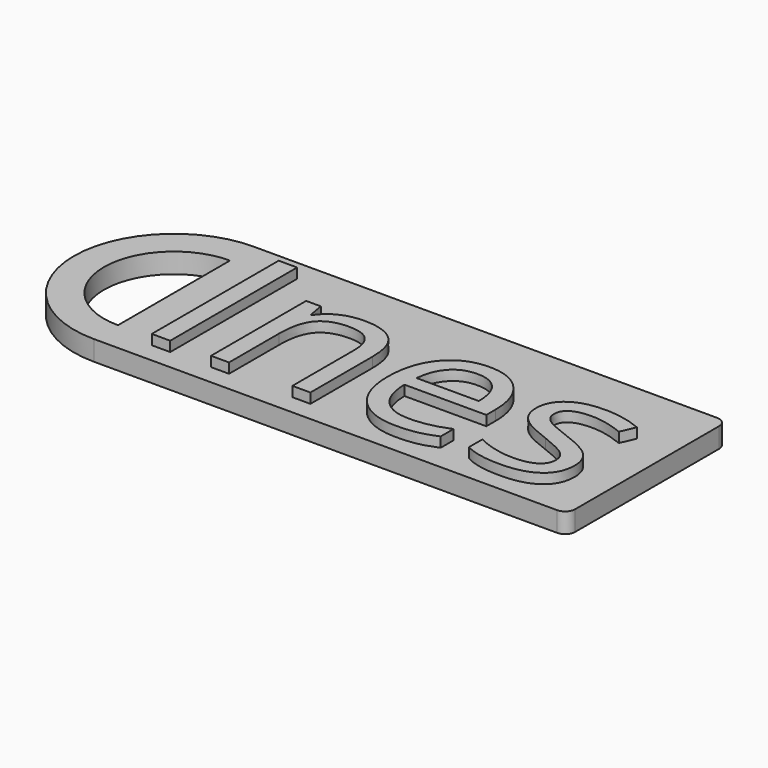
from build123d import *

# Parameters (mm, degrees)
F0_W         = 1.84375
F0_H         = 15.8645833333
F0_TEXT_SIZE = 22.2222222222
F1_DEPTH     = 2
F2_DEPTH     = 3
F3_R         = 1


# Not quite as in the source:
# - Text() gives the source's letters only with a copy of the font that has no kerning and outlines rounded to 1/6400 em; it was checked with that copy


with BuildPart() as f1:
    # F0 (on Top) → F1 (new body)
    with BuildSketch(Plane.XY):
        Polygon((28.77725482, 9.7942796086), (-18.5456618466, 9.7942796086), (-18.5456618466, 6.7942796086), (-18.5456618466, -7.2057203914), (-18.5456618466, -10.2057203914), (28.77725482, -10.2057203914), align=None)
        with Locations((-13.4432312911, -0.2734287247)):
            Rectangle(F0_W, F0_H, mode=Mode.SUBTRACT)
        with BuildLine():
            Line((1.4994770423, -8.2057203914), (-0.3026062911, -8.2057203914))
            Line((-0.3026062911, -8.2057203914), (-0.3026062911, -0.5112759469))
            add(Edge.make_bspline(
                [(-0.3026062911, -0.5112759469), (-0.3026062911, 0.940112942), (-0.9640646244, 1.6571268309)],
                knots=[0, 0, 0, 1, 1, 1], degree=2))
            add(Edge.make_bspline(
                [(-0.9640646244, 1.6571268309), (-1.6255229577, 2.3741407197), (-3.0387174022, 2.3741407197)],
                knots=[0, 0, 0, 1, 1, 1], degree=2))
            add(Edge.make_bspline(
                [(-3.0387174022, 2.3741407197), (-4.9033007355, 2.3741407197), (-5.7713562911, 1.3654601642)],
                knots=[0, 0, 0, 1, 1, 1], degree=2))
            add(Edge.make_bspline(
                [(-5.7713562911, 1.3654601642), (-6.6394118466, 0.3567796086), (-6.6394118466, -1.966137058)],
                knots=[0, 0, 0, 1, 1, 1], degree=2))
            Line((-6.6394118466, -1.966137058), (-6.6394118466, -8.2057203914))
            Line((-6.6394118466, -8.2057203914), (-8.44149518, -8.2057203914))
            Line((-8.44149518, -8.2057203914), (-8.44149518, 3.6866407197))
            Line((-8.44149518, 3.6866407197), (-6.9762174022, 3.6866407197))
            Line((-6.9762174022, 3.6866407197), (-6.6845507355, 2.0581684975))
            Line((-6.6845507355, 2.0581684975), (-6.59774518, 2.0581684975))
            add(Edge.make_bspline(
                [(-6.59774518, 2.0581684975), (-6.0421896244, 2.9366407197), (-5.0439257355, 3.4210157197)],
                knots=[0, 0, 0, 1, 1, 1], degree=2))
            add(Edge.make_bspline(
                [(-5.0439257355, 3.4210157197), (-4.0456618466, 3.9053907197), (-2.8199674022, 3.9053907197)],
                knots=[0, 0, 0, 1, 1, 1], degree=2))
            add(Edge.make_bspline(
                [(-2.8199674022, 3.9053907197), (-0.6706618466, 3.9053907197), (0.4144075978, 2.8689323864)],
                knots=[0, 0, 0, 1, 1, 1], degree=2))
            add(Edge.make_bspline(
                [(0.4144075978, 2.8689323864), (1.4994770423, 1.8324740531), (1.4994770423, -0.4487759469)],
                knots=[0, 0, 0, 1, 1, 1], degree=2))
            Line((1.4994770423, -0.4487759469), (1.4994770423, -8.2057203914))
        make_face(mode=Mode.SUBTRACT)
        with BuildLine():
            add(Edge.make_bspline(
                [(12.27725482, -8.2439148358), (11.4265603756, -8.4244703914), (10.2216992645, -8.4244703914)],
                knots=[0, 0, 0, 1, 1, 1], degree=2))
            add(Edge.make_bspline(
                [(10.2216992645, -8.4244703914), (7.5862825978, -8.4244703914), (6.0602409311, -6.8168315025)],
                knots=[0, 0, 0, 1, 1, 1], degree=2))
            add(Edge.make_bspline(
                [(6.0602409311, -6.8168315025), (4.5341992645, -5.2091926136), (4.5341992645, -2.3584981691)],
                knots=[0, 0, 0, 1, 1, 1], degree=2))
            add(Edge.make_bspline(
                [(4.5341992645, -2.3584981691), (4.5341992645, 0.5199740531), (5.9508659311, 2.2126823864)],
                knots=[0, 0, 0, 1, 1, 1], degree=2))
            add(Edge.make_bspline(
                [(5.9508659311, 2.2126823864), (7.3675325978, 3.9053907197), (9.7564214867, 3.9053907197)],
                knots=[0, 0, 0, 1, 1, 1], degree=2))
            add(Edge.make_bspline(
                [(9.7564214867, 3.9053907197), (11.9890603756, 3.9053907197), (13.2911437089, 2.4349046086)],
                knots=[0, 0, 0, 1, 1, 1], degree=2))
            add(Edge.make_bspline(
                [(13.2911437089, 2.4349046086), (14.5932270423, 0.9644184975), (14.5932270423, -1.4453037247)],
                knots=[0, 0, 0, 1, 1, 1], degree=2))
            Line((14.5932270423, -1.4453037247), (14.5932270423, -2.5841926136))
            Line((14.5932270423, -2.5841926136), (6.40225482, -2.5841926136))
            add(Edge.make_bspline(
                [(6.40225482, -2.5841926136), (6.4578103756, -4.6779426136), (7.4612825978, -5.763012058)],
                knots=[0, 0, 0, 1, 1, 1], degree=2))
            add(Edge.make_bspline(
                [(7.4612825978, -5.763012058), (8.46475482, -6.8480815025), (10.2876714867, -6.8480815025)],
                knots=[0, 0, 0, 1, 1, 1], degree=2))
            add(Edge.make_bspline(
                [(10.2876714867, -6.8480815025), (12.2078103756, -6.8480815025), (14.0828103756, -6.0459981691)],
                knots=[0, 0, 0, 1, 1, 1], degree=2))
            Line((14.0828103756, -6.0459981691), (14.0828103756, -7.653637058))
            add(Edge.make_bspline(
                [(14.0828103756, -7.653637058), (13.1279492645, -8.0633592803), (12.27725482, -8.2439148358)],
                knots=[0, 0, 0, 1, 1, 1], degree=2))
        make_face(mode=Mode.SUBTRACT)
        with BuildLine():
            add(Edge.make_bspline(
                [(24.5932270423, -2.997387058), (25.3362825978, -3.778637058), (25.3362825978, -4.9626648358)],
                knots=[0, 0, 0, 1, 1, 1], degree=2))
            add(Edge.make_bspline(
                [(25.3362825978, -4.9626648358), (25.3362825978, -6.622387058), (24.1001714867, -7.5234287247)],
                knots=[0, 0, 0, 1, 1, 1], degree=2))
            add(Edge.make_bspline(
                [(24.1001714867, -7.5234287247), (22.8640603756, -8.4244703914), (20.6279492645, -8.4244703914)],
                knots=[0, 0, 0, 1, 1, 1], degree=2))
            add(Edge.make_bspline(
                [(20.6279492645, -8.4244703914), (18.2633659311, -8.4244703914), (16.9404492645, -7.6744703914)],
                knots=[0, 0, 0, 1, 1, 1], degree=2))
            Line((16.9404492645, -7.6744703914), (16.9404492645, -6.0043315025))
            add(Edge.make_bspline(
                [(16.9404492645, -6.0043315025), (17.7980881534, -6.4383592803), (18.7789909311, -6.6866231691)],
                knots=[0, 0, 0, 1, 1, 1], degree=2))
            add(Edge.make_bspline(
                [(18.7789909311, -6.6866231691), (19.7598937089, -6.934887058), (20.6730881534, -6.934887058)],
                knots=[0, 0, 0, 1, 1, 1], degree=2))
            add(Edge.make_bspline(
                [(20.6730881534, -6.934887058), (22.0828103756, -6.934887058), (22.8414909311, -6.4852342803)],
                knots=[0, 0, 0, 1, 1, 1], degree=2))
            add(Edge.make_bspline(
                [(22.8414909311, -6.4852342803), (23.6001714867, -6.0355815025), (23.6001714867, -5.1119703914)],
                knots=[0, 0, 0, 1, 1, 1], degree=2))
            add(Edge.make_bspline(
                [(23.6001714867, -5.1119703914), (23.6001714867, -4.4175259469), (22.9994770423, -3.9244703914)],
                knots=[0, 0, 0, 1, 1, 1], degree=2))
            add(Edge.make_bspline(
                [(22.9994770423, -3.9244703914), (22.3987825978, -3.4314148358), (20.6487825978, -2.7578037247)],
                knots=[0, 0, 0, 1, 1, 1], degree=2))
            add(Edge.make_bspline(
                [(20.6487825978, -2.7578037247), (18.9890603756, -2.1397481691), (18.2894075978, -1.6779426136)],
                knots=[0, 0, 0, 1, 1, 1], degree=2))
            add(Edge.make_bspline(
                [(18.2894075978, -1.6779426136), (17.58975482, -1.216137058), (17.2477409311, -0.6310676136)],
                knots=[0, 0, 0, 1, 1, 1], degree=2))
            add(Edge.make_bspline(
                [(17.2477409311, -0.6310676136), (16.9057270423, -0.0459981691), (16.9057270423, 0.7665018309)],
                knots=[0, 0, 0, 1, 1, 1], degree=2))
            add(Edge.make_bspline(
                [(16.9057270423, 0.7665018309), (16.9057270423, 2.221362942), (18.08975482, 3.0633768309)],
                knots=[0, 0, 0, 1, 1, 1], degree=2))
            add(Edge.make_bspline(
                [(18.08975482, 3.0633768309), (19.2737825978, 3.9053907197), (21.3328103756, 3.9053907197)],
                knots=[0, 0, 0, 1, 1, 1], degree=2))
            add(Edge.make_bspline(
                [(21.3328103756, 3.9053907197), (23.2529492645, 3.9053907197), (25.08975482, 3.1241407197)],
                knots=[0, 0, 0, 1, 1, 1], degree=2))
            Line((25.08975482, 3.1241407197), (24.4473937089, 1.658862942))
            add(Edge.make_bspline(
                [(24.4473937089, 1.658862942), (22.6591992645, 2.3949740531), (21.2043381534, 2.3949740531)],
                knots=[0, 0, 0, 1, 1, 1], degree=2))
            add(Edge.make_bspline(
                [(21.2043381534, 2.3949740531), (19.9230881534, 2.3949740531), (19.2720464867, 1.9939323864)],
                knots=[0, 0, 0, 1, 1, 1], degree=2))
            add(Edge.make_bspline(
                [(19.2720464867, 1.9939323864), (18.62100482, 1.5928907197), (18.62100482, 0.8880296086)],
                knots=[0, 0, 0, 1, 1, 1], degree=2))
            add(Edge.make_bspline(
                [(18.62100482, 0.8880296086), (18.62100482, 0.408862942), (18.8657964867, 0.0737934975)],
                knots=[0, 0, 0, 1, 1, 1], degree=2))
            add(Edge.make_bspline(
                [(18.8657964867, 0.0737934975), (19.1105881534, -0.2612759469), (19.65225482, -0.5650953914)],
                knots=[0, 0, 0, 1, 1, 1], degree=2))
            add(Edge.make_bspline(
                [(19.65225482, -0.5650953914), (20.1939214867, -0.8689148358), (21.7355881534, -1.4453037247)],
                knots=[0, 0, 0, 1, 1, 1], degree=2))
            add(Edge.make_bspline(
                [(21.7355881534, -1.4453037247), (23.8501714867, -2.216137058), (24.5932270423, -2.997387058)],
                knots=[0, 0, 0, 1, 1, 1], degree=2))
        make_face(mode=Mode.SUBTRACT)
        with BuildLine():
            Line((-18.5456618466, 6.7942796086), (-18.5456618466, 9.7942796086))
            ThreePointArc((-18.5456618466, 9.7942796086), (-28.5456618466, -0.2057203914), (-18.5456618466, -10.2057203914))
            Line((-18.5456618466, -10.2057203914), (-18.5456618466, -7.2057203914))
            ThreePointArc((-18.5456618466, -7.2057203914), (-25.5456618466, -0.2057203914), (-18.5456618466, 6.7942796086))
        make_face()
        with Locations((-16.5456618466, -8.2057203914)):
            Text('Ines', F0_TEXT_SIZE, font='Open Sans', text_align=(TextAlign.LEFT, TextAlign.BOTTOM))
        with BuildLine():
            add(Edge.make_bspline(
                [(11.9039909311, 1.4887240531), (11.1453103756, 2.3949740531), (9.7321159311, 2.3949740531)],
                knots=[0, 0, 0, 1, 1, 1], degree=2))
            add(Edge.make_bspline(
                [(9.7321159311, 2.3949740531), (8.3015603756, 2.3949740531), (7.44912982, 1.4626823864)],
                knots=[0, 0, 0, 1, 1, 1], degree=2))
            add(Edge.make_bspline(
                [(7.44912982, 1.4626823864), (6.5966992645, 0.5303907197), (6.4439214867, -1.1189148358)],
                knots=[0, 0, 0, 1, 1, 1], degree=2))
            Line((6.4439214867, -1.1189148358), (12.6626714867, -1.1189148358))
            add(Edge.make_bspline(
                [(12.6626714867, -1.1189148358), (12.6626714867, 0.5824740531), (11.9039909311, 1.4887240531)],
                knots=[0, 0, 0, 1, 1, 1], degree=2))
        make_face()
    extrude(amount=F1_DEPTH)

    # F0 (on Top) → F2 (join)
    with BuildSketch(Plane.XY):
        with Locations((-16.5456618466, -8.2057203914)):
            Text('Ines', F0_TEXT_SIZE, font='Open Sans', text_align=(TextAlign.LEFT, TextAlign.BOTTOM))
    extrude(amount=F2_DEPTH)

    # F3
    f3_edges = [f1.edges().sort_by_distance(p)[0] for p in [
        (28.777255, 9.79428, 1),
        (28.777255, -10.20572, 1),
    ]]
    fillet(f3_edges, radius=F3_R)


solid = f1.part
